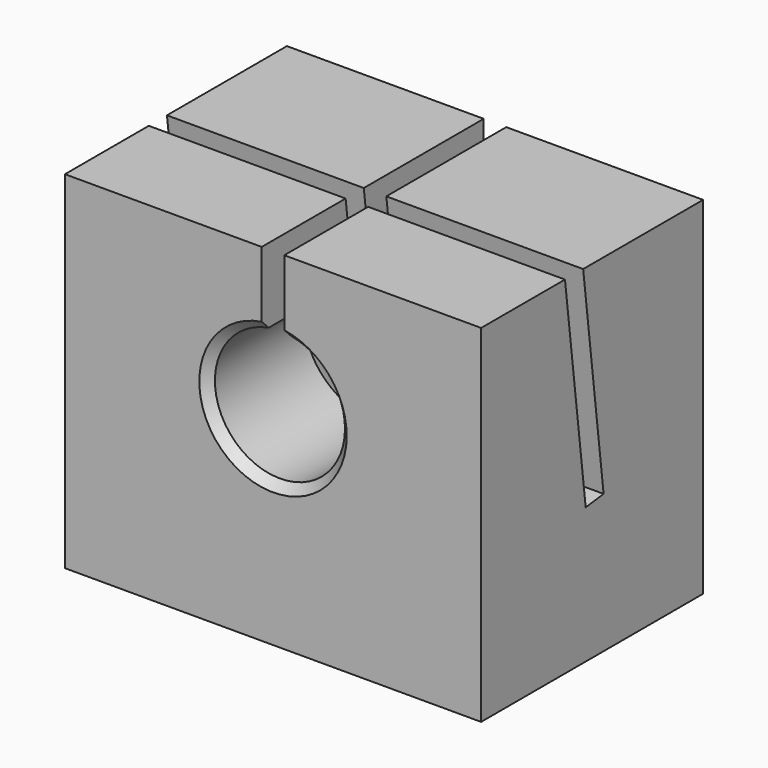
from build123d import *

# Parameters (mm, degrees)
F1_DEPTH = 8
F2_SIZE  = 0.25
F4_W     = 17.8603331085
F4_H     = 0.65
F5_DEPTH = 6.5


with BuildPart() as f1:
    # F0 (on Front) → F1 (new body)
    with BuildSketch(Plane.XZ):
        with BuildLine():
            Line((-24.4284769839, 17.7468117975), (-30.1034769839, 17.7468117975))
            Line((-30.1034769839, 17.7468117975), (-30.1034769839, 7.7468117975))
            Line((-30.1034769839, 7.7468117975), (-18.1034769839, 7.7468117975))
            Line((-18.1034769839, 7.7468117975), (-18.1034769839, 17.7468117975))
            Line((-18.1034769839, 17.7468117975), (-23.7784769839, 17.7468117975))
            Line((-23.7784769839, 17.7468117975), (-23.7784769839, 15.5934303288))
            ThreePointArc((-23.7784769839, 15.5934303288), (-22.6673363223, 14.9522681427), (-22.2284769839, 13.7468117975))
            ThreePointArc((-22.2284769839, 13.7468117975), (-25.308933329, 12.3106711359), (-24.4284769839, 15.5934303288))
            Line((-24.4284769839, 15.5934303288), (-24.4284769839, 17.7468117975))
        make_face()
    extrude(amount=F1_DEPTH)

    # F2
    f2_edges = [f1.edges().sort_by_distance(p)[0] for p in [
        (-24.103477, 0, 11.871812),
        (-24.103477, -8, 11.871812),
    ]]
    chamfer(f2_edges, length=F2_SIZE)

    # F4 (on face) → F5 (cut)
    with BuildSketch(Plane(origin=(0, -2.2654882704, 18.4509213023), x_dir=(1, 0, 0), z_dir=(0, 0.1218693434, -0.9925461516))):
        with Locations((-24.4247596711, 2.4525769118)):
            Rectangle(F4_W, F4_H)
    extrude(amount=F5_DEPTH, mode=Mode.SUBTRACT)


solid = f1.part
